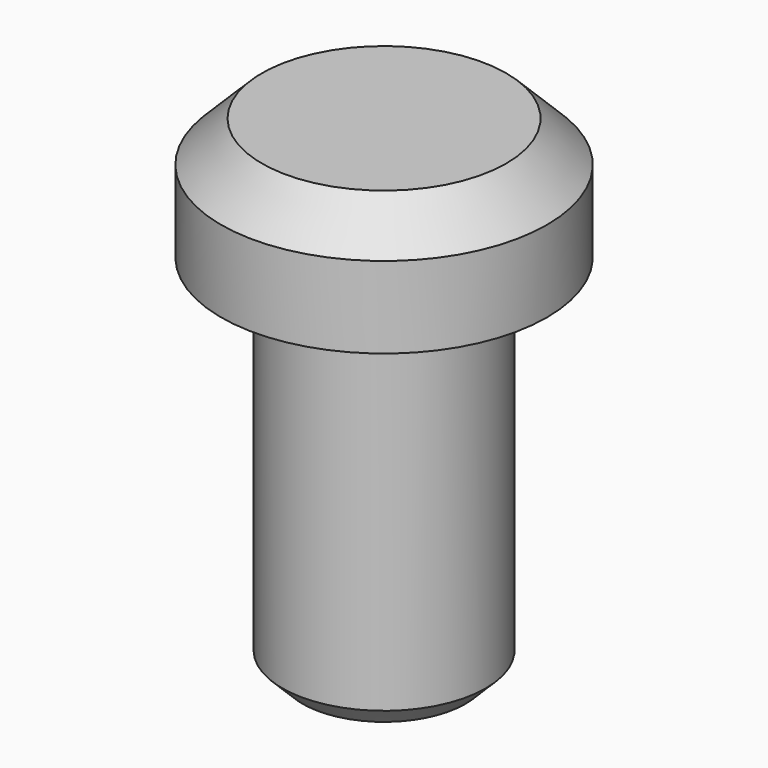
from build123d import *

# Parameters (mm, degrees)
F0_R     = 40
F1_DEPTH = 10
F3_SIZE  = 9.99999
F2_R     = 40
F4_DEPTH = 20
F5_R     = 25
F6_DEPTH = 90
F7_SIZE  = 5


# Not quite as in the source:
# - a fillet or chamfer is up to 0.001 mm smaller than in the source, because OpenCascade refuses the exact size


with BuildPart() as f1:
    # F0 (on Top) → F1 (new body)
    with BuildSketch(Plane.XY):
        Circle(F0_R)
    extrude(amount=F1_DEPTH)

    # F3 (size 10 in the source; OpenCascade refuses exactly that, so slightly less here)
    f3_edges = [f1.edges().sort_by_distance(p)[0] for p in [
        (-40, 0, 10),
    ]]
    chamfer(f3_edges, length=F3_SIZE)

    # F2 (on face) → F4 (join)
    with BuildSketch(Plane(origin=(0, 0, 0), x_dir=(1, 0, 0), z_dir=(0, 0, -1))):
        Circle(F2_R)
    extrude(amount=F4_DEPTH)

    # F5 (on face) → F6 (join)
    with BuildSketch(Plane(origin=(0, 0, -20), x_dir=(1, 0, 0), z_dir=(0, 0, -1))):
        Circle(F5_R)
    extrude(amount=F6_DEPTH)

    # F7
    f7_edges = [f1.edges().sort_by_distance(p)[0] for p in [
        (-25, 0, -110),
    ]]
    chamfer(f7_edges, length=F7_SIZE)


solid = f1.part
